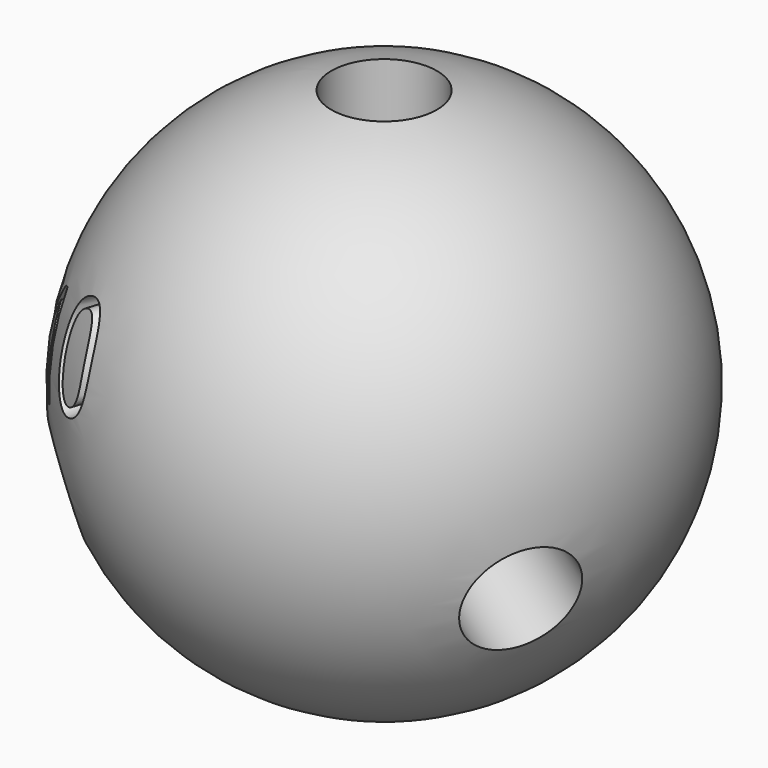
from build123d import *

# Parameters (mm, degrees)
F5_R          = 3.175
F6_DEPTH      = 50.8
F8_ANGLE      = 106.2
F9_ANGLE      = 115.9
F10_ANGLE     = 110
F12_TEXT_SIZE = 4.9149491436
F13_DEPTH     = 25.4
F15_TEXT_SIZE = 7.2365329187
F16_DEPTH     = 25.4


# Not quite as in the source:
# - a length typed as a fraction of an inch, garbled in the dataset ("3 / 203.2 mm" for 3/8 in), is restored
# - Text() gives the source's letters only with a copy of the font that has no kerning and outlines rounded to 1/6400 em; it was checked with that copy


with BuildPart() as f2:
    # F0 (on Front) → F2 (revolve)
    with BuildSketch(Plane.XZ):
        with BuildLine():
            Line((0, -15.875), (0, 15.875))
            ThreePointArc((0, 15.875), (-15.875, 0), (0, -15.875))
        make_face()
    revolve(axis=Axis((0, 0, 0), (0, 0, 1)))

    # F12 (on offset) → F13 (cut)
    with BuildSketch(Plane(origin=(0, 29.8795380298, -8.6808082644), x_dir=(-1, 0, 0), z_dir=(0, 0.9602936857, -0.278991106))):
        with Locations((-6.3070369042, 3.3637222368)):
            Text('106.2', F12_TEXT_SIZE, font='Open Sans', text_align=(TextAlign.LEFT, TextAlign.BOTTOM))
    extrude(amount=-F13_DEPTH, mode=Mode.SUBTRACT)

    # F15 (on offset) → F16 (cut)
    with BuildSketch(Plane(origin=(-21.4572820242, -20.7935528712, -8.6808082644), x_dir=(0.6195036195, -0.7439092375, 0.2506278351), z_dir=(-0.6896121493, -0.6682806643, -0.278991106))):
        with Locations((-4.8539401032, 4.1269222274)):
            Text('110', F15_TEXT_SIZE, font='Open Sans', text_align=(TextAlign.LEFT, TextAlign.BOTTOM))
    extrude(amount=-F16_DEPTH, mode=Mode.SUBTRACT)


with BuildPart() as f6:
    # F5 (on offset) → F6 (new body)
    with BuildSketch(Plane.XY.offset(5.715)):
        Circle(F5_R)
    extrude(amount=F6_DEPTH)


with BuildPart() as f8_1:
    # F8: copy of F6
    add(f6.part.rotate(Axis((-31.9024734199, 0, 0), (-1, 0, 0)), F8_ANGLE))


with BuildPart() as f9_1:
    # F9: copy of F8_1
    add(f8_1.part.rotate(Axis((0, 0, -26.9088633358), (0, 0, -1)), F9_ANGLE))


with BuildPart() as f10_1:
    # F10: copy of F9_1
    add(f9_1.part.rotate(Axis((0, 0, -26.9088633358), (0, 0, -1)), F10_ANGLE))


with BuildPart() as f2_1:
    add(f2.part)

    # F17: cut F6, F8_1, F10_1, F9_1
    add(f6.part, mode=Mode.SUBTRACT)
    add(f8_1.part, mode=Mode.SUBTRACT)
    add(f10_1.part, mode=Mode.SUBTRACT)
    add(f9_1.part, mode=Mode.SUBTRACT)


solid = f2_1.part
